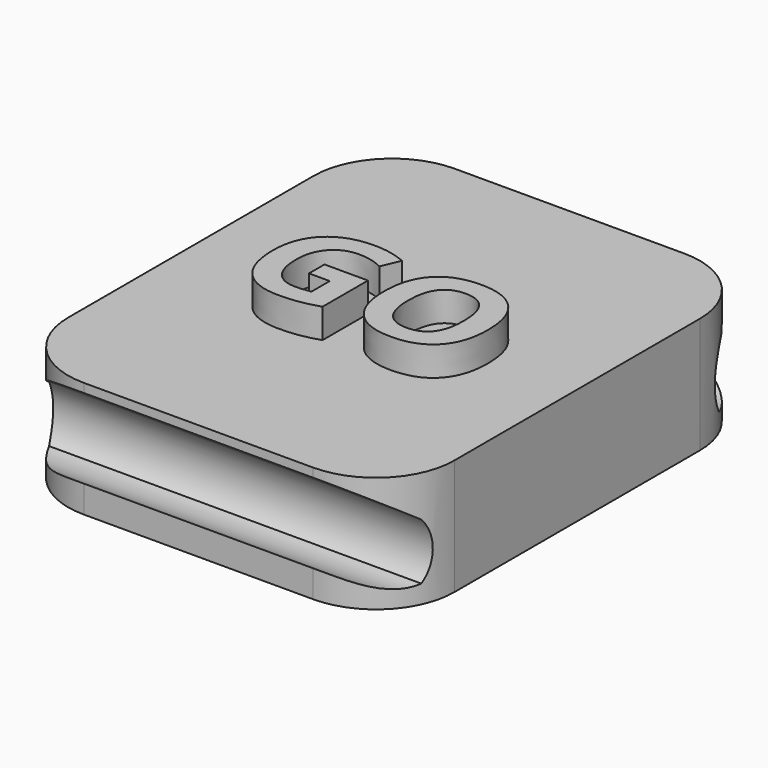
from build123d import *

# Parameters (mm, degrees)
F0_W         = 25
F0_H         = 30
F1_DEPTH     = 7.5
F3_DEPTH     = 25.4
F4_T1_DEPTH  = 25.9770765059
F4_T3_DEPTH  = 27.1628476489
F5_W         = 10.7245780528
F5_H         = 2.6884500403
F6_DEPTH     = 1.524
F7_R         = 0.635
F8_TEXT_SIZE = 9.9228746775
F9_DEPTH     = 1.905


# Not quite as in the source:
# - a fillet or chamfer that OpenCascade refuses, or shapes differently, is made with other operations: its cross-section is extruded or revolved along the edge and cut away or added
# - Text() gives the source's letters only with a copy of the font that has no kerning and outlines rounded to 1/6400 em; it was checked with that copy


with BuildPart() as f1:
    # F0 (on Top) → F1 (new body)
    with BuildSketch(Plane.XY):
        with Locations((12.5, 15)):
            Rectangle(F0_W, F0_H)
    extrude(amount=F1_DEPTH)

    # F2 (on face) → F3 (cut)
    with BuildSketch(Plane.YZ.offset(25)):
        with BuildLine():
            Line((0, 6.9229234941), (0, 1.7628476489))
            ThreePointArc((0, 1.7628476489), (1.4221317574, 1.1558507525), (2.9680202715, 1.1895059142))
            ThreePointArc((2.9680202715, 1.1895059142), (3.5975132946, 3.0151467072), (2.9680202715, 4.8407875001))
            Line((2.9680202715, 4.8407875001), (0, 6.9229234941))
        make_face()
        with BuildLine():
            Line((30, 6.9229234941), (27.0319797285, 4.8407875001))
            ThreePointArc((27.0319797285, 4.8407875001), (26.4024867054, 3.0151467072), (27.0319797285, 1.1895059142))
            ThreePointArc((27.0319797285, 1.1895059142), (28.5778682426, 1.1558507525), (30, 1.7628476489))
            Line((30, 1.7628476489), (30, 6.9229234941))
        make_face()
    extrude(amount=-F3_DEPTH, mode=Mode.SUBTRACT)

    # F4: fillet of radius 5.08 on 8 edges, made by hand

    # F4_s2 → F4_t1 (cut)
    with BuildSketch(Plane.XY.offset(-5.7770765059)):
        with BuildLine():
            ThreePointArc((19.92, 0), (23.5121024484, 1.4878975516), (25, 5.08))
            Line((25, 5.08), (25, 0))
            Line((25, 0), (19.92, 0))
        make_face()
        with BuildLine():
            ThreePointArc((0, 5.08), (1.4878975516, 1.4878975516), (5.08, 0))
            Line((5.08, 0), (0, 0))
            Line((0, 0), (0, 5.08))
        make_face()
        with BuildLine():
            ThreePointArc((0, 24.92), (1.4878975516, 28.5121024484), (5.08, 30))
            Line((5.08, 30), (0, 30))
            Line((0, 30), (0, 24.92))
        make_face()
        with BuildLine():
            ThreePointArc((19.92, 30), (23.5121024484, 28.5121024484), (25, 24.92))
            Line((25, 24.92), (25, 30))
            Line((25, 30), (19.92, 30))
        make_face()
    extrude(amount=F4_T1_DEPTH, mode=Mode.SUBTRACT)

    # F4_s4 → F4_t3 (cut)
    with BuildSketch(Plane.XY.offset(-12.7)):
        with BuildLine():
            ThreePointArc((0, 5.08), (1.4878975516, 1.4878975516), (5.08, 0))
            Line((5.08, 0), (0, 0))
            Line((0, 0), (0, 5.08))
        make_face()
        with BuildLine():
            ThreePointArc((0, 24.92), (1.4878975516, 28.5121024484), (5.08, 30))
            Line((5.08, 30), (0, 30))
            Line((0, 30), (0, 24.92))
        make_face()
        with BuildLine():
            ThreePointArc((19.92, 0), (23.5121024484, 1.4878975516), (25, 5.08))
            Line((25, 5.08), (25, 0))
            Line((25, 0), (19.92, 0))
        make_face()
        with BuildLine():
            ThreePointArc((19.92, 30), (23.5121024484, 28.5121024484), (25, 24.92))
            Line((25, 24.92), (25, 30))
            Line((25, 30), (19.92, 30))
        make_face()
    extrude(amount=F4_T3_DEPTH, mode=Mode.SUBTRACT)

    # F5 (on face) → F6 (join)
    with BuildSketch(Plane(origin=(0, 0, 0), x_dir=(0, -1, 0), z_dir=(-1, 0, 0))):
        with Locations((-15.1792485267, 3.8743120385)):
            Rectangle(F5_W, F5_H)
    extrude(amount=F6_DEPTH)

    # F7
    f7_edges = [f1.edges().sort_by_distance(p)[0] for p in [
        (-0.762, 9.81696, 5.218537),
        (-0.762, 9.81696, 2.530087),
        (-0.762, 20.541538, 5.218537),
        (-0.762, 20.541538, 2.530087),
    ]]
    fillet(f7_edges, radius=F7_R)

    # F8 (on face) → F9 (join)
    with BuildSketch(Plane.XY.offset(7.5)):
        with Locations((5.1886630245, 10.8732394874)):
            Text('GO', F8_TEXT_SIZE, font='Open Sans', font_style=FontStyle.BOLD, text_align=(TextAlign.LEFT, TextAlign.BOTTOM))
    extrude(amount=F9_DEPTH)


solid = f1.part
